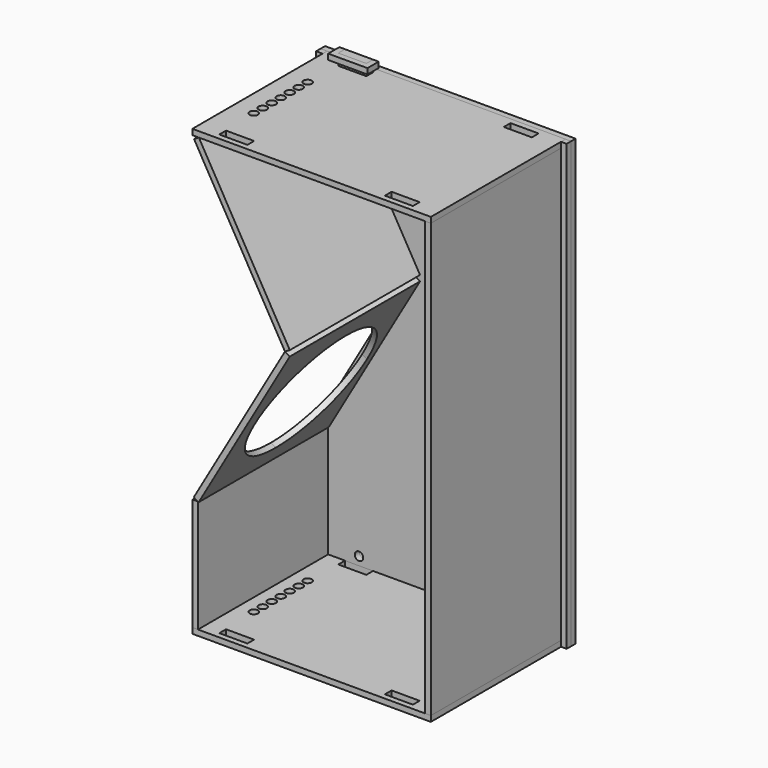
from build123d import *

# Parameters (mm, degrees)
F7_DEPTH       = 30
F7_DEPTH_BACK  = 30
F1_W           = 2
F1_H           = 154.4626819264
F8_DEPTH       = 30
F8_DEPTH_BACK  = 30
F9_DEPTH       = 30
F9_DEPTH_BACK  = 30
F10_DEPTH      = 30
F10_DEPTH_BACK = 30
F1_H_2         = 40.1473286269
F11_DEPTH      = 30
F11_DEPTH_BACK = 30
F12_DEPTH      = 30
F12_DEPTH_BACK = 30
F13_DEPTH      = 25
F14_R          = 1.5
F14_W          = 10
F14_H          = 3
F15_DEPTH      = 2
F16_W          = 10
F16_H          = 3
F16_R          = 1.5
F17_DEPTH      = 2
F18_DEPTH      = 2
F5_W           = 2
F5_H           = 158.4626819264
F19_DEPTH      = 2
F20_DEPTH      = 2
F22_W          = 10
F22_H          = 3
F23_DEPTH      = 12
F23_DEPTH_BACK = 2
F24_DEPTH      = 2
F25_R          = 2
F26_R          = 1.5
F27_DEPTH      = 50


# Not quite as in the source:
# - a feature names something its author has since deleted; it is built from what else it names


with BuildPart() as f7:
    # F1 (on Front) → F7 (new body, two sides)
    with BuildSketch(Plane.XZ) as f7_sk:
        Polygon((-4, 109.3871500693), (-4, 107.3871500693), (-1.6905989232, 107.3871500693), (79, 107.3871500693), (81, 107.3871500693), (81, 109.3871500693), align=None)
    extrude(amount=F7_DEPTH)
    extrude(f7_sk.sketch, amount=-F7_DEPTH_BACK)

    # F14 (on face) → F15 (cut)
    with BuildSketch(Plane.XY.offset(109.3871500693)):
        with Locations((3.5, 12)):
            Circle(F14_R)
        with Locations((3.5, 8)):
            Circle(F14_R)
        with Locations((3.5, 4)):
            Circle(F14_R)
        with Locations((3.5, -4)):
            Circle(F14_R)
        with Locations((3.5, 0)):
            Circle(F14_R)
        with Locations((3.5, -8)):
            Circle(F14_R)
        with Locations((3.5, -12)):
            Circle(F14_R)
        with Locations((9, 26.5)):
            Rectangle(F14_W, F14_H)
        with Locations((68, 26.5)):
            Rectangle(F14_W, F14_H)
        with Locations((68, -26.5)):
            Rectangle(F14_W, F14_H)
        with Locations((9, -26.5)):
            Rectangle(F14_W, F14_H)
    extrude(amount=-F15_DEPTH, mode=Mode.SUBTRACT)


with BuildPart() as f8:
    # F1 (on Front) → F8 (new body, two sides)
    with BuildSketch(Plane.XZ) as f8_sk:
        with Locations((80, 30.1558091061)):
            Rectangle(F1_W, F1_H)
    extrude(amount=F8_DEPTH)
    extrude(f8_sk.sketch, amount=-F8_DEPTH_BACK)


with BuildPart() as f9:
    # F1 (on Front) → F9 (new body, two sides)
    with BuildSketch(Plane.XZ) as f9_sk:
        Polygon((-3.4226497308, 106.3871500693), (29, 50.2294734195), (30.7320508076, 51.2294734195), (-1.6905989232, 107.3871500693), align=None)
    extrude(amount=F9_DEPTH)
    extrude(f9_sk.sketch, amount=-F9_DEPTH_BACK)


with BuildPart() as f10:
    # F1 (on Front) → F10 (new body, two sides)
    with BuildSketch(Plane.XZ) as f10_sk:
        Polygon((25, 43.3012701892), (0, 0), (-3.5, -6.0621778265), (-2, -6.9282032303), (-1.7679491924, -7.0621778265), (30.7320508076, 49.2294734195), (29, 50.2294734195), align=None)
    extrude(amount=F10_DEPTH)
    extrude(f10_sk.sketch, amount=-F10_DEPTH_BACK)

    # F4 (on line) → F13 (cut)
    with BuildSketch(Plane(origin=(0, 0, 0), x_dir=(0, 1, 0), z_dir=(0.8660254038, 0, -0.5))):
        with BuildLine():
            Line((0, 50), (0, 0))
            ThreePointArc((0, 0), (17.6776695297, 7.3223304703), (25, 25))
            ThreePointArc((25, 25), (17.6776695297, 42.6776695297), (0, 50))
        make_face()
        with BuildLine():
            ThreePointArc((0, 50), (-25, 25), (0, 0))
            Line((0, 0), (0, 50))
        make_face()
    extrude(amount=F13_DEPTH, mode=Mode.SUBTRACT)


with BuildPart() as f11:
    # F1 (on Front) → F11 (new body, two sides)
    with BuildSketch(Plane.XZ) as f11_sk:
        with Locations((-3, -27.0018675437)):
            Rectangle(F1_W, F1_H_2)
    extrude(amount=F11_DEPTH)
    extrude(f11_sk.sketch, amount=-F11_DEPTH_BACK)


with BuildPart() as f12:
    # F1 (on Front) → F12 (new body, two sides)
    with BuildSketch(Plane.XZ) as f12_sk:
        Polygon((-2, -47.0755318572), (-4, -47.0755318572), (-4, -49.0755318572), (81, -49.0755318572), (81, -47.0755318572), (79, -47.0755318572), align=None)
    extrude(amount=F12_DEPTH)
    extrude(f12_sk.sketch, amount=-F12_DEPTH_BACK)

    # F16 (on face) → F17 (cut)
    with BuildSketch(Plane(origin=(0, 0, -49.0755318572), x_dir=(1, 0, 0), z_dir=(0, 0, -1))):
        with Locations((9, -26.5)):
            Rectangle(F16_W, F16_H)
        with Locations((3.5, -12)):
            Circle(F16_R)
        with Locations((3.5, -8)):
            Circle(F16_R)
        with Locations((3.5, -4)):
            Circle(F16_R)
        with Locations((3.5, 0)):
            Circle(F16_R)
        with Locations((3.5, 4)):
            Circle(F16_R)
        with Locations((3.5, 8)):
            Circle(F16_R)
        with Locations((3.5, 12)):
            Circle(F16_R)
        with Locations((9, 26.5)):
            Rectangle(F16_W, F16_H)
        with Locations((68, 26.5)):
            Rectangle(F16_W, F16_H)
        with Locations((68, -26.5)):
            Rectangle(F16_W, F16_H)
    extrude(amount=-F17_DEPTH, mode=Mode.SUBTRACT)


with BuildPart() as f18:
    # F5 (on offset) → F18 (new body)
    with BuildSketch(Plane.XZ.offset(-30)):
        Polygon((-2, -6.9282032303), (-2, -47.0755318572), (79, -47.0755318572), (79, 107.3871500693), (-1.6905989232, 107.3871500693), (30.7320508076, 51.2294734195), (29, 50.2294734195), (30.7320508076, 49.2294734195), (-1.7679491924, -7.0621778265), align=None)
    extrude(amount=F18_DEPTH)


with BuildPart() as f19:
    # F5 (on offset) → F19 (new body)
    with BuildSketch(Plane.XZ.offset(-30)):
        with Locations((82, 30.1558091061)):
            Rectangle(F5_W, F5_H)
    extrude(amount=F19_DEPTH)


with BuildPart() as f19b:
    # F5 (on offset) → F19, piece 2 (new body)
    with BuildSketch(Plane.XZ.offset(-30)):
        Polygon((25, 43.3012701892), (29, 50.2294734195), (-4, 107.3871500693), (-4, 109.3871500693), (-6.3094010768, 109.3871500693), (-6.3094010768, 107.3871500693), (26.6905989232, 50.2294734195), (-6, -6.3923048454), (-6, -49.0755318572), (-4, -49.0755318572), (-4, -47.0755318572), (-4, -6.9282032303), (0, 0), align=None)
    extrude(amount=F19_DEPTH)


with BuildPart() as f20:
    # F6 (on offset) → F20 (new body)
    with BuildSketch(Plane.XZ.offset(-30)):
        Polygon((-4, -49.0755318572), (81, -49.0755318572), (83, -49.0755318572), (83, 109.3871500693), (81, 109.3871500693), (-4, 109.3871500693), (-6.3094010768, 109.3871500693), (-6.3094010768, 107.3871500693), (26.6905989232, 50.2294734195), (-6, -6.3923048454), (-6, -49.0755318572), align=None)
    extrude(amount=-F20_DEPTH)


with BuildPart() as f23:
    # F22 (on offset) → F23 (new body, two sides)
    with BuildSketch(Plane.XY.offset(111.3871500693)) as f23_sk:
        with Locations((9, 26.5)):
            Rectangle(F22_W, F22_H)
    extrude(amount=-F23_DEPTH)
    extrude(f23_sk.sketch, amount=F23_DEPTH_BACK)

    # F25
    f25_edges = [f23.edges().sort_by_distance(p)[0] for p in [
        (14, 26.5, 99.38715),
        (4, 26.5, 99.38715),
    ]]
    fillet(f25_edges, radius=F25_R)


with BuildPart() as f24:
    # F22 (on offset) → F24 (new body)
    with BuildSketch(Plane.XY.offset(111.3871500693)):
        Polygon((14, 28), (14, 25), (4, 25), (4, 28), (2, 28), (2, 23), (16, 23), (16, 28), align=None)
    extrude(amount=F24_DEPTH)


with BuildPart() as f27_tool:
    # F26 (on face) → F27 (new body)
    with BuildSketch(Plane.XZ.offset(-25)):
        with Locations((9, 104.3871500693)):
            Circle(F26_R)
        with Locations((68.3094010768, 104.3871500693)):
            Circle(F26_R)
        with Locations((9, -44.0755318572)):
            Circle(F26_R)
        with Locations((68.3094010768, -44.0755318572)):
            Circle(F26_R)
    extrude(amount=-F27_DEPTH)


with BuildPart() as f18_1:
    add(f18.part)

    # F27: cut by f27_tool
    add(f27_tool.part, mode=Mode.SUBTRACT)


with BuildPart() as f20_1:
    add(f20.part)

    # F27: cut by f27_tool
    add(f27_tool.part, mode=Mode.SUBTRACT)


with BuildPart() as f23_1:
    add(f23.part)

    # F27: cut by f27_tool
    add(f27_tool.part, mode=Mode.SUBTRACT)


solid = Compound([f7.part, f8.part, f9.part, f10.part, f11.part, f12.part, f19.part, f19b.part, f24.part, f18_1.part, f20_1.part, f23_1.part])
